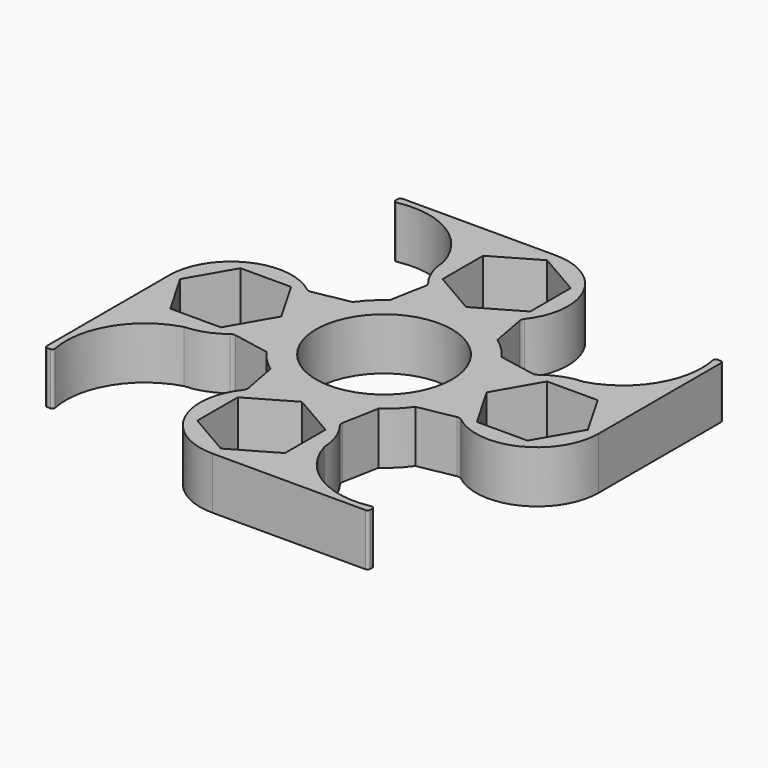
from build123d import *

# Parameters (mm, degrees)
F0_R     = 11.075
F2_DEPTH = 8.5
F3_COUNT = 4


# Not quite as in the source:
# - a feature names something its author has since deleted; it is built from what else it names


with BuildPart() as f2:
    # F0 (on Top) → F2 (new body)
    with BuildSketch(Plane.XY):
        with BuildLine():
            Line((-7.6826518036, 18.0394667333), (-8.7891866596, 12.1552539201))
            ThreePointArc((-8.7891866596, 12.1552539201), (0, -15), (8.7891866596, 12.1552539201))
            Line((8.7891866596, 12.1552539201), (7.6826518036, 18.0394667333))
            ThreePointArc((7.6826518036, 18.0394667333), (7.6938199579, 18.4608846247), (7.8776597121, 18.840253458))
            ThreePointArc((7.8776597121, 18.840253458), (8.9888115293, 29.3819250667), (0, 35))
            Line((0, 35), (-25, 35))
            ThreePointArc((-25, 35), (-25.2828427125, 34.8828427125), (-25.4, 34.6))
            Line((-25.4, 34.6), (-25.4, 34.1))
            ThreePointArc((-25.4, 34.1), (-25.2534392204, 33.7905350399), (-24.9211571922, 33.7078472088))
            ThreePointArc((-24.9211571922, 33.7078472088), (-15.6786460864, 32.0797048321), (-9.9925313497, 24.6135841297))
            ThreePointArc((-9.9925313497, 24.6135841297), (-9.3898226238, 21.5603443352), (-7.8776597121, 18.840253458))
            ThreePointArc((-7.8776597121, 18.840253458), (-7.6938199579, 18.4608846247), (-7.6826518036, 18.0394667333))
        make_face()
        Circle(F0_R, mode=Mode.SUBTRACT)
        Polygon((0, 33.2561088494), (7.15, 29.1280544247), (7.15, 20.8719455753), (0, 16.7438911506), (-7.15, 20.8719455753), (-7.15, 29.1280544247), align=None, mode=Mode.SUBTRACT)
    extrude(amount=F2_DEPTH)

    # F3: F2 ×4 about axis
    f3_axis = Axis((0, 0, 16.6777409613), (0, 0, 1))


with BuildPart() as f2_1:
    add(f2.part)
    for i in range(1, F3_COUNT):
        add(f2.part.rotate(f3_axis, i * 360 / F3_COUNT))


solid = f2_1.part
